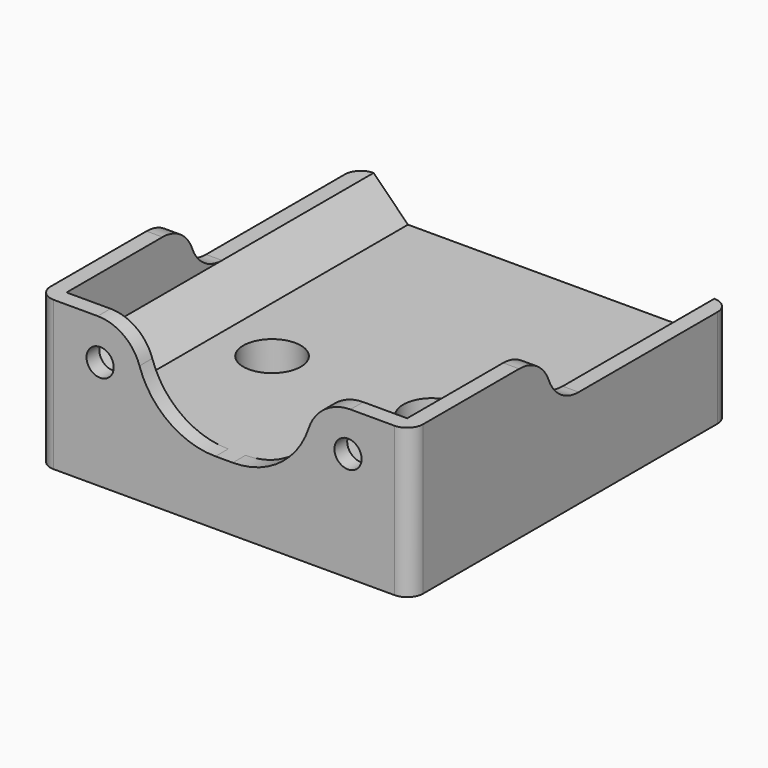
from build123d import *

# Parameters (mm, degrees)
F1_DEPTH     = 24
F2_R         = 1.7
F3_DEPTH     = 2
F4_R         = 5.5
F5_T1_DEPTH  = 2
F6_W         = 2
F6_H         = 6.35
F7_DEPTH     = 20
F8_R         = 5
F9_T4_DEPTH  = 2
F9_T9_DEPTH  = 12.7751879692
F9_T15_DEPTH = 2
F9_T20_DEPTH = 2
F9_T25_DEPTH = 2
F9_T30_DEPTH = 12.7751879692
F10_R        = 2.2
F11_DEPTH    = 8
F10_R_2      = 3.6
F12_DEPTH    = 4
F13_R        = 1
F14_DEPTH    = 3.6
F15_R        = 2


# Not quite as in the source:
# - a fillet or chamfer that OpenCascade refuses, or shapes differently, is made with other operations: its cross-section is extruded or revolved along the edge and cut away or added


with BuildPart() as f1:
    # F0 (on Front) → F1 (new body, symmetric)
    with BuildSketch(Plane.XZ):
        Polygon((-23.3, 12.3), (-23.3, 0), (0, 0), (23.3, 0), (23.3, 12.3), (21.3, 12.3), (17, 8), (0, 8), (-17, 8), (-21.3, 12.3), align=None)
    extrude(amount=F1_DEPTH, both=True)

    # F2 (on face) → F3 (join)
    with BuildSketch(Plane.XZ.offset(24)):
        Polygon((-23.3, 18.65), (-23.3, 12.3), (-21.3, 12.3), (-17, 8), (-10.3, 8), (-10.3, 18.65), align=None)
        with Locations((-15.5, 13.65)):
            Circle(F2_R, mode=Mode.SUBTRACT)
        Polygon((21.3, 12.3), (23.3, 12.3), (23.3, 18.65), (10.3, 18.65), (10.3, 8), (17, 8), align=None)
        with Locations((15.5, 13.65)):
            Circle(F2_R, mode=Mode.SUBTRACT)
        Polygon((-21.3, 12.3), (-23.3, 12.3), (-23.3, 0), (23.3, 0), (23.3, 12.3), (21.3, 12.3), (17, 8), (10.3, 8), (-10.3, 8), (-17, 8), align=None)
    extrude(amount=F3_DEPTH)

    # F4
    f4_edges = [f1.edges().sort_by_distance(p)[0] for p in [
        (-10.3, -25, 18.65),
        (10.3, -25, 18.65),
    ]]
    fillet(f4_edges, radius=F4_R)

    # F5: fillet of radius 10 on 2 edges, made by hand

    # F5_s2 → F5_t1 (join)
    with BuildSketch(Plane.XZ.offset(24)):
        with BuildLine():
            ThreePointArc((-1.0783322956, 8), (-6.9396323825, 9.8978298407), (-10.5761824275, 14.8709677419))
            Line((-10.5761824275, 14.8709677419), (-11.5259674406, 14.5580645161))
            ThreePointArc((-11.5259674406, 14.5580645161), (-11.3, 13.15), (-11.3, 8))
            Line((-11.3, 8), (-10.3, 7))
            Line((-10.3, 7), (-1.0783322956, 7))
            Line((-1.0783322956, 7), (-1.0783322956, 8))
        make_face()
        with BuildLine():
            ThreePointArc((10.5761824275, 14.8709677419), (6.9396323825, 9.8978298407), (1.0783322956, 8))
            Line((1.0783322956, 8), (1.0783322956, 7))
            Line((1.0783322956, 7), (10.3, 7))
            Line((10.3, 7), (11.3, 8))
            ThreePointArc((11.3, 8), (11.3, 13.15), (11.5259674406, 14.5580645161))
            Line((11.5259674406, 14.5580645161), (10.5761824275, 14.8709677419))
        make_face()
    extrude(amount=F5_T1_DEPTH)

    # F6 (on face) → F7 (join)
    with BuildSketch(Plane(origin=(0, -24, 0), x_dir=(-1, 0, 0), z_dir=(0, 1, 0))):
        with Locations((-22.3, 15.475)):
            Rectangle(F6_W, F6_H)
        with Locations((22.3, 15.475)):
            Rectangle(F6_W, F6_H)
    extrude(amount=F7_DEPTH)

    # F8
    f8_edges = [f1.edges().sort_by_distance(p)[0] for p in [
        (22.3, -4, 18.65),
        (-22.3, -4, 18.65),
    ]]
    fillet(f8_edges, radius=F8_R)

    # F9: fillet of radius 5 on 2 edges, made by hand


with BuildPart() as f9_tool2:
    # F9_s3 → F9_t4 (new body)
    with BuildSketch(Plane.YZ.offset(-21.3)):
        with BuildLine():
            ThreePointArc((-4.3449624062, 15.475), (-2.5072817297, 13.1693220895), (0.3100751877, 12.3))
            Line((0.3100751877, 12.3), (0.3100751877, 11.8))
            Line((0.3100751877, 11.8), (-4, 11.8))
            Line((-4, 11.8), (-4.5, 12.3))
            ThreePointArc((-4.5, 12.3), (-4.5, 13.65), (-4.8104661656, 15.2925))
            Line((-4.8104661656, 15.2925), (-4.3449624062, 15.475))
        make_face()
    extrude(amount=-F9_T4_DEPTH)

    split(bisect_by=Plane(origin=(-4.5, 0, -4.5), x_dir=(0, 1, 0), z_dir=(0.7071067812, 0, 0.7071067812)), keep=Keep.TOP)


with BuildPart() as f1_1:
    add(f1.part)

    # F9_t1: union F9_tool2
    add(f9_tool2.part)


with BuildPart() as f9_tool7:
    # F9_s8 → F9_t9 (new body)
    with BuildSketch(Plane.YZ.offset(-10.5248120308)):
        with BuildLine():
            ThreePointArc((-4.3449624062, 15.475), (-2.5072817297, 13.1693220895), (0.3100751877, 12.3))
            Line((0.3100751877, 12.3), (0.3100751877, 11.8))
            Line((0.3100751877, 11.8), (-4, 11.8))
            Line((-4, 11.8), (-4.5, 12.3))
            ThreePointArc((-4.5, 12.3), (-4.5, 13.65), (-4.8104661656, 15.2925))
            Line((-4.8104661656, 15.2925), (-4.3449624062, 15.475))
        make_face()
    extrude(amount=-F9_T9_DEPTH)

    split(bisect_by=Plane.YZ.offset(-21.3), keep=Keep.TOP)

    split(bisect_by=Plane(origin=(-4.5, 0, -4.5), x_dir=(0, 1, 0), z_dir=(-0.7071067812, 0, -0.7071067812)), keep=Keep.TOP)


with BuildPart() as f1_2:
    add(f1_1.part)

    # F9_t6: union F9_tool7
    add(f9_tool7.part)


with BuildPart() as f9_tool13:
    # F9_s14 → F9_t15 (new body)
    with BuildSketch(Plane.YZ.offset(-21.3)):
        with BuildLine():
            ThreePointArc((-4.3449624062, 15.475), (-2.5072817297, 13.1693220895), (0.3100751877, 12.3))
            Line((0.3100751877, 12.3), (0.3100751877, 11.8))
            Line((0.3100751877, 11.8), (-4, 11.8))
            Line((-4, 11.8), (-4.5, 12.3))
            ThreePointArc((-4.5, 12.3), (-4.5, 13.65), (-4.8104661656, 15.2925))
            Line((-4.8104661656, 15.2925), (-4.3449624062, 15.475))
        make_face()
    extrude(amount=-F9_T15_DEPTH)

    split(bisect_by=Plane(origin=(-4.5, 0, -4.5), x_dir=(0, 1, 0), z_dir=(-0.7071067812, 0, -0.7071067812)), keep=Keep.TOP)


with BuildPart() as f1_3:
    add(f1_2.part)

    # F9_t12: union F9_tool13
    add(f9_tool13.part)


with BuildPart() as f9_tool18:
    # F9_s19 → F9_t20 (new body)
    with BuildSketch(Plane.YZ.offset(23.3)):
        with BuildLine():
            ThreePointArc((0.3100751877, 12.3), (-2.5072817297, 13.1693220895), (-4.3449624062, 15.475))
            Line((-4.3449624062, 15.475), (-4.8104661656, 15.2925))
            ThreePointArc((-4.8104661656, 15.2925), (-4.5, 13.65), (-4.5, 12.3))
            Line((-4.5, 12.3), (-4, 11.8))
            Line((-4, 11.8), (0.3100751877, 11.8))
            Line((0.3100751877, 11.8), (0.3100751877, 12.3))
        make_face()
    extrude(amount=-F9_T20_DEPTH)

    split(bisect_by=Plane(origin=(4.5, 0, -4.5), x_dir=(0, 1, 0), z_dir=(0.7071067812, 0, -0.7071067812)), keep=Keep.TOP)


with BuildPart() as f1_4:
    add(f1_3.part)

    # F9_t17: union F9_tool18
    add(f9_tool18.part)


with BuildPart() as f9_tool23:
    # F9_s24 → F9_t25 (new body)
    with BuildSketch(Plane.YZ.offset(23.3)):
        with BuildLine():
            ThreePointArc((0.3100751877, 12.3), (-2.5072817297, 13.1693220895), (-4.3449624062, 15.475))
            Line((-4.3449624062, 15.475), (-4.8104661656, 15.2925))
            ThreePointArc((-4.8104661656, 15.2925), (-4.5, 13.65), (-4.5, 12.3))
            Line((-4.5, 12.3), (-4, 11.8))
            Line((-4, 11.8), (0.3100751877, 11.8))
            Line((0.3100751877, 11.8), (0.3100751877, 12.3))
        make_face()
    extrude(amount=-F9_T25_DEPTH)

    split(bisect_by=Plane(origin=(4.5, 0, -4.5), x_dir=(0, 1, 0), z_dir=(-0.7071067812, 0, 0.7071067812)), keep=Keep.TOP)


with BuildPart() as f1_5:
    add(f1_4.part)

    # F9_t22: union F9_tool23
    add(f9_tool23.part)


with BuildPart() as f9_tool28:
    # F9_s29 → F9_t30 (new body)
    with BuildSketch(Plane.YZ.offset(23.3)):
        with BuildLine():
            ThreePointArc((0.3100751877, 12.3), (-2.5072817297, 13.1693220895), (-4.3449624062, 15.475))
            Line((-4.3449624062, 15.475), (-4.8104661656, 15.2925))
            ThreePointArc((-4.8104661656, 15.2925), (-4.5, 13.65), (-4.5, 12.3))
            Line((-4.5, 12.3), (-4, 11.8))
            Line((-4, 11.8), (0.3100751877, 11.8))
            Line((0.3100751877, 11.8), (0.3100751877, 12.3))
        make_face()
    extrude(amount=-F9_T30_DEPTH)

    split(bisect_by=Plane(origin=(4.5, 0, -4.5), x_dir=(0, 1, 0), z_dir=(0.7071067812, 0, -0.7071067812)), keep=Keep.TOP)

    split(bisect_by=Plane.YZ.offset(21.3), keep=Keep.BOTTOM)


with BuildPart() as f1_6:
    add(f1_5.part)

    # F9_t27: union F9_tool28
    add(f9_tool28.part)

    # F10 (on face) → F11 (cut)
    with BuildSketch(Plane.XY.offset(8)):
        with Locations((10, -6)):
            Circle(F10_R)
        with Locations((-10, -6)):
            Circle(F10_R)
    extrude(amount=-F11_DEPTH, mode=Mode.SUBTRACT)

    # F10 (on face) → F12 (cut)
    with BuildSketch(Plane.XY.offset(8)):
        with Locations((10, -6)):
            Circle(F10_R_2)
        with Locations((10, -6)):
            Circle(F10_R, mode=Mode.SUBTRACT)
        with Locations((-10, -6)):
            Circle(F10_R_2)
        with Locations((-10, -6)):
            Circle(F10_R, mode=Mode.SUBTRACT)
    extrude(amount=-F12_DEPTH, mode=Mode.SUBTRACT)

    # F13 (on face) → F14 (cut)
    with BuildSketch(Plane(origin=(0, 0, 0), x_dir=(1, 0, 0), z_dir=(0, 0, -1))):
        with Locations((6.116718427, 3.178630789)):
            Circle(F13_R)
        with Locations((6.116718427, 8.821369211)):
            Circle(F13_R)
        with Locations((11.483281573, 10.5650712782)):
            Circle(F13_R)
        with Locations((11.483281573, 1.4349287218)):
            Circle(F13_R)
        with Locations((14.8, 6)):
            Circle(F13_R)
        with Locations((-11.483281573, 10.5650712782)):
            Circle(F13_R)
        with Locations((-14.8, 6)):
            Circle(F13_R)
        with Locations((-11.483281573, 1.4349287218)):
            Circle(F13_R)
        with Locations((-6.116718427, 3.178630789)):
            Circle(F13_R)
        with Locations((-6.116718427, 8.821369211)):
            Circle(F13_R)
    extrude(amount=-F14_DEPTH, mode=Mode.SUBTRACT)

    # F15
    f15_edges = [f1_6.edges().sort_by_distance(p)[0] for p in [
        (-23.3, 24, 6.15),
        (23.3, 24, 6.15),
        (-23.3, -26, 9.325),
        (23.3, -26, 9.325),
    ]]
    fillet(f15_edges, radius=F15_R)


solid = f1_6.part
